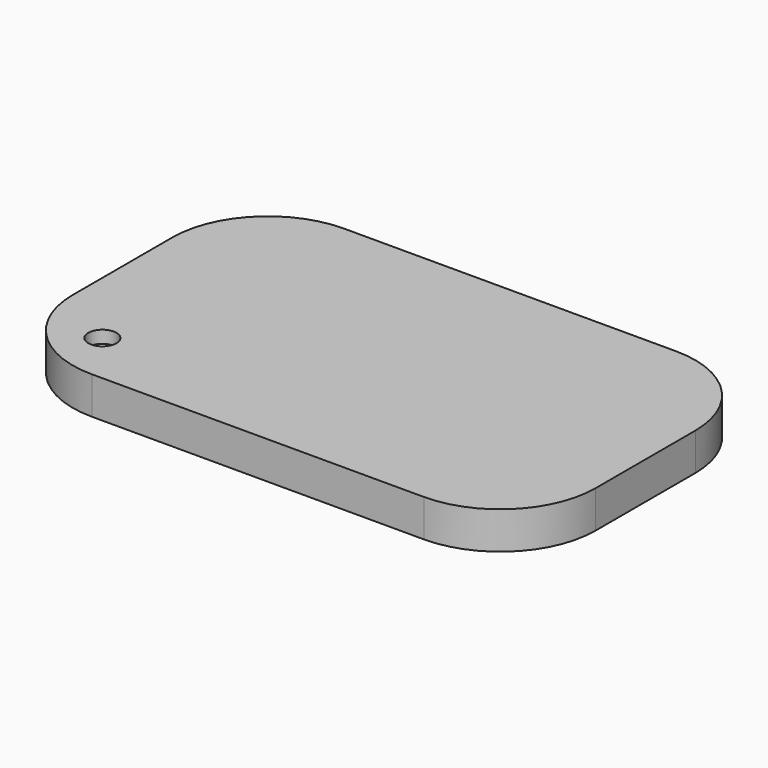
from build123d import *

# Parameters (mm, degrees)
F0_W         = 60
F0_H         = 35
F1_DEPTH     = 3
F2_R         = 10
F3_T         = 1.5
F4_TEXT_SIZE = 11.1111111111
F5_DEPTH     = 1.5
F7_D         = 3.4


# Not quite as in the source:
# - Text() gives the source's letters only with a copy of the font that has no kerning and outlines rounded to 1/6400 em; it was checked with that copy


with BuildPart() as f1:
    # F0 (on Top) → F1 (new body)
    with BuildSketch(Plane.XY):
        Rectangle(F0_W, F0_H)
    extrude(amount=F1_DEPTH)

    # F2
    f2_edges = [f1.edges().sort_by_distance(p)[0] for p in [
        (30, 17.5, 1.5),
        (-30, -17.5, 1.5),
        (30, -17.5, 1.5),
        (-30, 17.5, 1.5),
    ]]
    fillet(f2_edges, radius=F2_R)

    # F3
    f3_openings = [f1.faces().sort_by_distance(p)[0] for p in [
        (0, 0, 0),
    ]]
    offset(amount=F3_T, openings=f3_openings, kind=Kind.INTERSECTION)

    # F4 (on face) → F5 (join)
    with BuildSketch(Plane(origin=(0, 0, 3), x_dir=(1, 0, 0), z_dir=(0, 0, -1))):
        with Locations((-21.6701388889, 2)):
            Text('GARAGE', F4_TEXT_SIZE, font='Open Sans', text_align=(TextAlign.LEFT, TextAlign.BOTTOM))
        with Locations((-15.1736111111, -10)):
            Text('LINKS', F4_TEXT_SIZE, font='Open Sans', text_align=(TextAlign.LEFT, TextAlign.BOTTOM))
    extrude(amount=F5_DEPTH)

    # F7 (through all)
    with Locations(Plane(origin=(0, 0, 3), x_dir=(1, 0, 0), z_dir=(0, 0, -1))):
        with Locations((-23.8400995731, 12.6071702689)):
            Hole(F7_D / 2)


solid = f1.part
